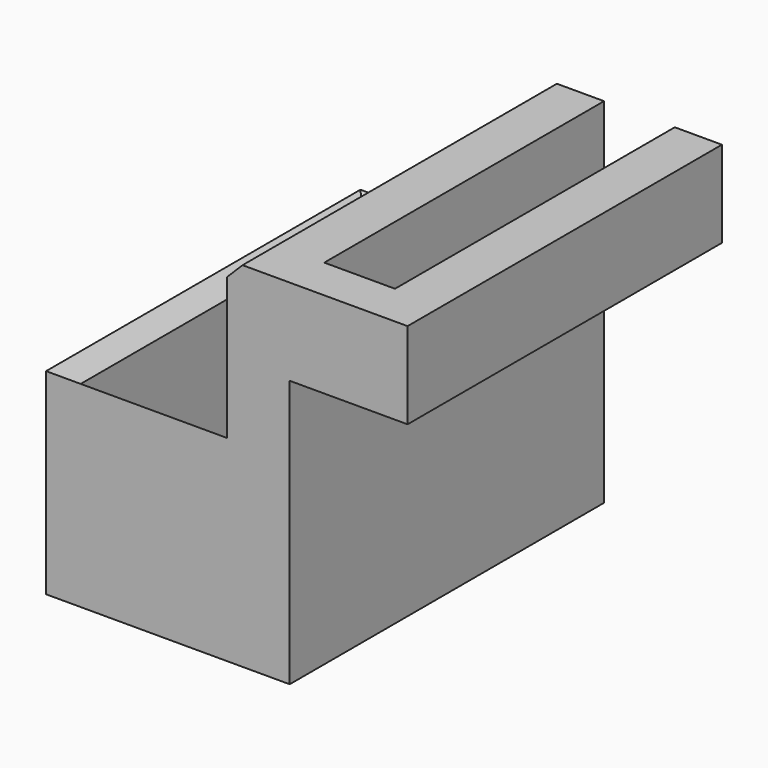
from build123d import *

# Parameters (mm, degrees)
F1_DEPTH = 25
F0_W     = 21
F0_H     = 46
F2_DEPTH = 2
F3_W     = 8
F3_H     = 50
F4_DEPTH = 20
F5_W     = 5.5
F5_H     = 11
F6_DEPTH = 15
F7_W     = 6
F7_H     = 11
F8_DEPTH = 44.5
F9_SIZE  = 1.99999


# Not quite as in the source:
# - a fillet or chamfer is up to 0.001 mm smaller than in the source, because OpenCascade refuses the exact size


with BuildPart() as f1:
    # F0 (on Top) → F1 (new body)
    with BuildSketch(Plane.XY):
        Polygon((0, 25), (0, 23), (0, -23), (0, -25), (8, -25), (8, 25), align=None)
        Polygon((-21, 23), (0, 23), (0, 25), (-23, 25), (-23, -25), (0, -25), (0, -23), (-21, -23), align=None)
    extrude(amount=F1_DEPTH)

    # F0 (on Top) → F2 (join)
    with BuildSketch(Plane.XY):
        Polygon((0, 25), (0, 23), (0, -23), (0, -25), (8, -25), (8, 25), align=None)
        with Locations((-10.5, 0)):
            Rectangle(F0_W, F0_H)
        Polygon((-21, 23), (0, 23), (0, 25), (-23, 25), (-23, -25), (0, -25), (0, -23), (-21, -23), align=None)
    extrude(amount=F2_DEPTH)

    # F3 (on face) → F4 (join)
    with BuildSketch(Plane.XY.offset(25)):
        with Locations((4, 0)):
            Rectangle(F3_W, F3_H)
    extrude(amount=F4_DEPTH)

    # F5 (on face) → F6 (join)
    with BuildSketch(Plane.YZ.offset(8)):
        with Locations((-22.25, 39.5)):
            Rectangle(F5_W, F5_H)
    extrude(amount=F6_DEPTH)

    # F7 (on face) → F8 (join, through all)
    with BuildSketch(Plane(origin=(0, -19.5, 0), x_dir=(-1, 0, 0), z_dir=(0, 1, 0))):
        with Locations((-20, 39.5)):
            Rectangle(F7_W, F7_H)
    extrude(amount=F8_DEPTH)

    # F9 (size 2 in the source; OpenCascade refuses exactly that, so slightly less here)
    f9_edges = [f1.edges().sort_by_distance(p)[0] for p in [
        (-10.5, 23, 25),
        (-21, 0, 25),
        (-10.5, -23, 25),
        (0, 0, 45),
    ]]
    chamfer(f9_edges, length=F9_SIZE)


solid = f1.part
